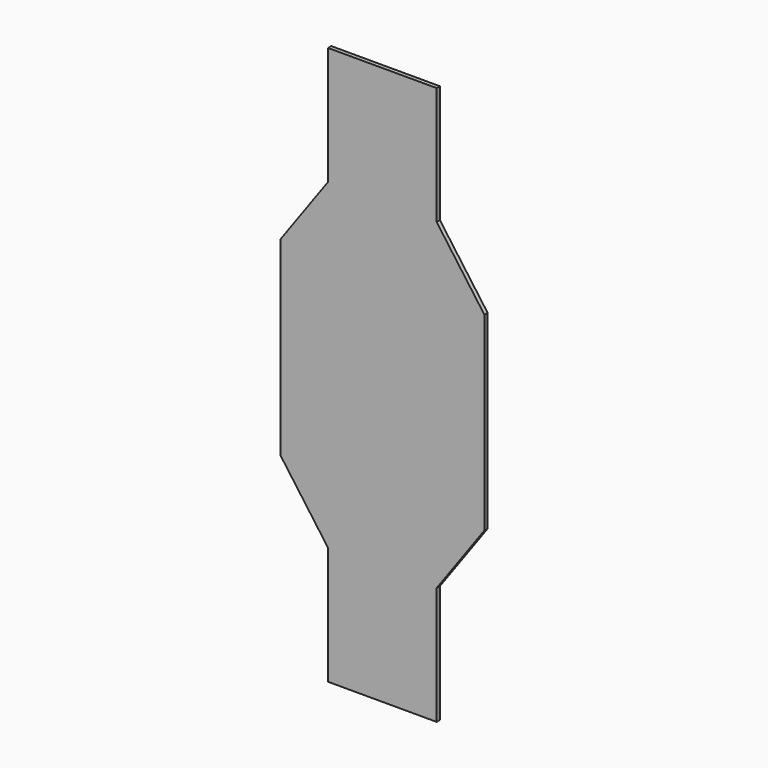
from build123d import *

# Parameters (mm, degrees)
F1_DEPTH = 19.05


# Not quite as in the source:
# - the program builds the solid bodies; features that only make, move or delete a surface that nothing else refers to are left out


with BuildPart() as f1:
    # F0 (on Front) → F1 (new body)
    with BuildSketch(Plane.XZ):
        Polygon((-515.5588388443, -1148.3222827911), (-515.5588388443, -2037.3222827911), (-292.5681887819, -2346.2497337966), (-292.5681887819, -2897.7202328353), (215.4318112181, -2897.7202328353), (215.4318112181, -2346.2497337966), (438.4224612806, -2037.3222827911), (438.4224612806, -1148.3222827911), (215.4318112181, -839.3948317857), (215.4318112181, -287.924332747), (-292.5681887819, -287.924332747), (-292.5681887819, -839.3948317857), align=None)
    extrude(amount=F1_DEPTH)


solid = f1.part
